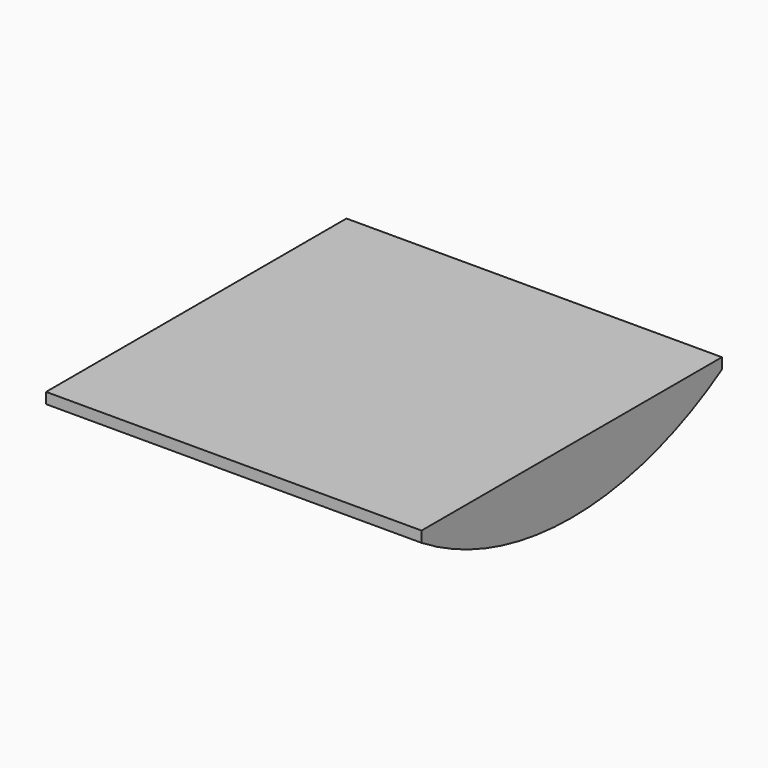
from build123d import *

# Parameters (mm, degrees)
F1_DEPTH = 25.4
F2_W     = 692.8203314
F2_H     = 692.8203314
F3_DEPTH = 20
F5_DEPTH = 20


# Not quite as in the source:
# - ends of sketch curves that miss each other by under 0.0002 mm in the source are joined


with BuildPart() as f1:
    # F0 (on Right) → F1 (new body)
    with BuildSketch(Plane.YZ):
        with BuildLine():
            Line((346.4101615138, -550), (-346.4101615138, -550))
            ThreePointArc((-346.4101615138, -550), (0, -650), (346.4101615138, -550))
        make_face()
    extrude(amount=F1_DEPTH)

    # F2 (on face) → F3 (join)
    with BuildSketch(Plane.XY.offset(-550)):
        with Locations((-321.0101657, -4.1862e-06)):
            Rectangle(F2_W, F2_H)
        Polygon((0, -346.4101615138), (0, 346.4101615138), (-667.4203314, 346.4101615138), (-667.4203314, -346.4101698862), align=None)
    extrude(amount=F3_DEPTH)


with BuildPart() as f5:
    # F4 (on face) → F5 (new body)
    with BuildSketch(Plane(origin=(-667.4203314, 0, 0), x_dir=(0, -1, 0), z_dir=(-1, 0, 0))):
        with BuildLine():
            Line((346.4101698862, -550), (-346.4101615138, -550))
            ThreePointArc((-346.4101615138, -550), (3.5422e-06, -650), (346.4101698862, -550))
        make_face()
    extrude(amount=-F5_DEPTH)


solid = Compound([f1.part, f5.part])
